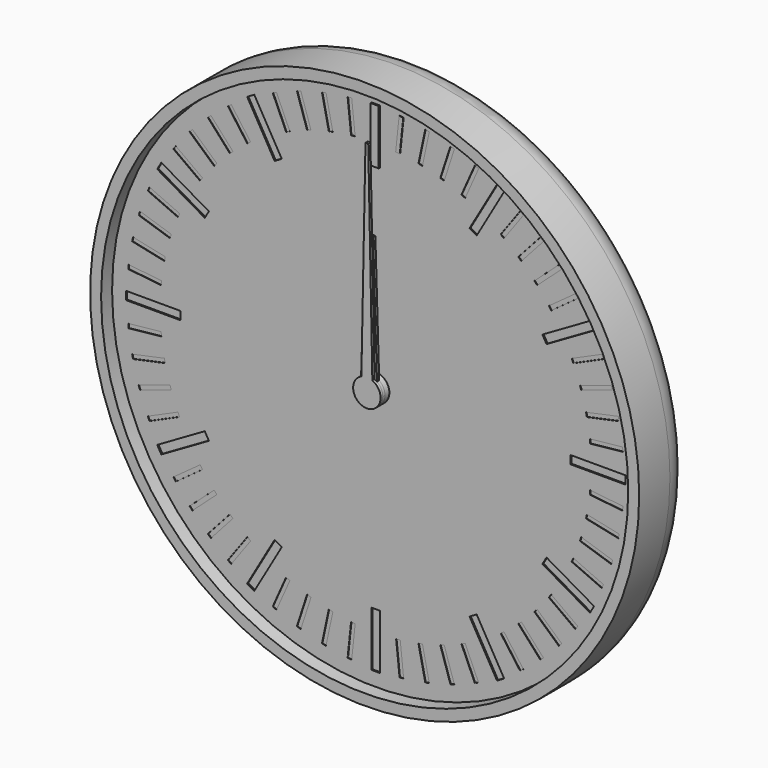
from build123d import *

# Parameters (mm, degrees)
F0_R      = 100
F1_DEPTH  = 24
F2_R      = 10
F3_T      = -4
F4_R      = 5
F4_R_2    = 3
F5_DEPTH  = 2
F6_DEPTH  = 19
F7_DEPTH  = 8
F9_DEPTH  = 4
F11_DEPTH = 4
F12_R     = 5
F12_R_2   = 3
F13_DEPTH = 2
F14_R     = 3
F15_DEPTH = 4
F17_DEPTH = 4
F18_R     = 3
F19_DEPTH = 2
F20_R     = 98
F20_R_2   = 5
F21_DEPTH = 1
F23_R     = 5
F23_R_2   = 3
F24_DEPTH = 2
F25_W     = 3
F25_H     = 20
F25_W_2   = 20
F25_H_2   = 3
F26_DEPTH = 0.5
F27_W     = 1.5
F27_H     = 12
F27_W_2   = 12
F27_H_2   = 1.5
F28_DEPTH = 0.2
F29_DEPTH = 1
F30_DEPTH = 0.4
F31_R     = 5
F31_R_2   = 3
F32_DEPTH = 5
F33_R     = 3
F34_DEPTH = 1
F36_DEPTH = 1


with BuildPart() as f1:
    # F0 (on Front) → F1 (new body)
    with BuildSketch(Plane.XZ):
        Circle(F0_R)
    extrude(amount=F1_DEPTH)

    # F2
    f2_edges = [f1.edges().sort_by_distance(p)[0] for p in [
        (-100, 0, 0),
    ]]
    fillet(f2_edges, radius=F2_R)

    # F3
    f3_openings = [f1.faces().sort_by_distance(p)[0] for p in [
        (0, -24, 0),
    ]]
    offset(amount=F3_T, openings=f3_openings)

    # F4 (on face) → F5 (join)
    with BuildSketch(Plane.XZ.offset(4)):
        Circle(F4_R)
        Circle(F4_R_2, mode=Mode.SUBTRACT)
        with Locations((40, 0)):
            Circle(F4_R)
        with Locations((40, 0)):
            Circle(F4_R_2, mode=Mode.SUBTRACT)
    extrude(amount=F5_DEPTH)


with BuildPart() as f6:
    # F6 (new): a face of the model
    f6_faces = [f1.part.faces().sort_by_distance(p)[0] for p in [
        (0, -4, 0),
    ]]
    extrude(f6_faces, amount=F6_DEPTH)

    # F8 (on face) → F9 (join)
    with BuildSketch(Plane.XZ.offset(6)):
        with BuildLine():
            ThreePointArc((9.2729637667, -1.3794085621), (9.3494561423, -0.6915886375), (9.375, 0))
            ThreePointArc((9.375, 0), (9.3494561423, 0.6915886375), (9.2729637667, 1.3794085621))
            ThreePointArc((9.2729637667, 1.3794085621), (8.9161548403, 2.8970343223), (8.3127812852, 4.3345463782))
            ThreePointArc((8.3127812852, 4.3345463782), (7.5845343223, 5.5104867402), (6.6911892658, 6.566476316))
            ThreePointArc((6.6911892658, 6.566476316), (5.5104867402, 7.5845343223), (4.1773988938, 8.3928519278))
            ThreePointArc((4.1773988938, 8.3928519278), (2.8970343223, 8.9161548403), (1.5536078905, 9.2453733036))
            ThreePointArc((1.5536078905, 9.2453733036), (0, 9.375), (-1.5536078905, 9.2453733036))
            ThreePointArc((-1.5536078905, 9.2453733036), (-2.8970343223, 8.9161548403), (-4.1773988938, 8.3928519278))
            ThreePointArc((-4.1773988938, 8.3928519278), (-5.5104867402, 7.5845343223), (-6.6911892658, 6.566476316))
            ThreePointArc((-6.6911892658, 6.566476316), (-7.5845343223, 5.5104867402), (-8.3127812852, 4.3345463782))
            ThreePointArc((-8.3127812852, 4.3345463782), (-8.9161548403, 2.8970343223), (-9.2729637667, 1.3794085621))
            ThreePointArc((-9.2729637667, 1.3794085621), (-9.375, 0), (-9.2729637667, -1.3794085621))
            ThreePointArc((-9.2729637667, -1.3794085621), (-8.9161548403, -2.8970343223), (-8.3127812852, -4.3345463782))
            ThreePointArc((-8.3127812852, -4.3345463782), (-7.5845343223, -5.5104867402), (-6.6911892658, -6.566476316))
            ThreePointArc((-6.6911892658, -6.566476316), (-5.5104867402, -7.5845343223), (-4.1773988938, -8.3928519278))
            ThreePointArc((-4.1773988938, -8.3928519278), (-2.8970343223, -8.9161548403), (-1.5536078905, -9.2453733036))
            ThreePointArc((-1.5536078905, -9.2453733036), (0, -9.375), (1.5536078905, -9.2453733036))
            ThreePointArc((1.5536078905, -9.2453733036), (2.8970343223, -8.9161548403), (4.1773988938, -8.3928519278))
            ThreePointArc((4.1773988938, -8.3928519278), (5.5104867402, -7.5845343223), (6.6911892658, -6.566476316))
            ThreePointArc((6.6911892658, -6.566476316), (7.5845343223, -5.5104867402), (8.3127812852, -4.3345463782))
            ThreePointArc((8.3127812852, -4.3345463782), (8.9161548403, -2.8970343223), (9.2729637667, -1.3794085621))
        make_face()
        with BuildLine():
            ThreePointArc((8.3127812852, 4.3345463782), (8.9161548403, 2.8970343223), (9.2729637667, 1.3794085621))
            Line((9.2729637667, 1.3794085621), (11.1823199426, 2.3946312492))
            Line((11.1823199426, 2.3946312492), (10.8182678729, 3.515068311))
            Line((10.8182678729, 3.515068311), (10.4542158031, 4.6355053728))
            Line((10.4542158031, 4.6355053728), (8.3127812852, 4.3345463782))
        make_face()
        with BuildLine():
            Line((11.1823199426, -2.3946312492), (9.2729637667, -1.3794085621))
            ThreePointArc((9.2729637667, -1.3794085621), (8.9161548403, -2.8970343223), (8.3127812852, -4.3345463782))
            Line((8.3127812852, -4.3345463782), (10.4542158031, -4.6355053728))
            Line((10.4542158031, -4.6355053728), (10.8182678729, -3.515068311))
            Line((10.8182678729, -3.515068311), (11.1823199426, -2.3946312492))
        make_face()
        with BuildLine():
            ThreePointArc((4.1773988938, 8.3928519278), (5.5104867402, 7.5845343223), (6.6911892658, 6.566476316))
            Line((6.6911892658, 6.566476316), (7.6391579371, 8.5101001246))
            Line((7.6391579371, 8.5101001246), (6.6860572448, 9.202568311))
            Line((6.6860572448, 9.202568311), (5.7329565525, 9.8950364974))
            Line((5.7329565525, 9.8950364974), (4.1773988938, 8.3928519278))
        make_face()
        with BuildLine():
            Line((7.6391579371, -8.5101001246), (6.6911892658, -6.566476316))
            ThreePointArc((6.6911892658, -6.566476316), (5.5104867402, -7.5845343223), (4.1773988938, -8.3928519278))
            Line((4.1773988938, -8.3928519278), (5.7329565525, -9.8950364974))
            Line((5.7329565525, -9.8950364974), (6.6860572448, -9.202568311))
            Line((6.6860572448, -9.202568311), (7.6391579371, -8.5101001246))
        make_face()
        with BuildLine():
            ThreePointArc((-1.5536078905, 9.2453733036), (0, 9.375), (1.5536078905, 9.2453733036))
            Line((1.5536078905, 9.2453733036), (1.1780972451, 11.375))
            Line((1.1780972451, 11.375), (0, 11.375))
            Line((0, 11.375), (-1.1780972451, 11.375))
            Line((-1.1780972451, 11.375), (-1.5536078905, 9.2453733036))
        make_face()
        with BuildLine():
            Line((1.1780972451, -11.375), (1.5536078905, -9.2453733036))
            ThreePointArc((1.5536078905, -9.2453733036), (0, -9.375), (-1.5536078905, -9.2453733036))
            Line((-1.5536078905, -9.2453733036), (-1.1780972451, -11.375))
            Line((-1.1780972451, -11.375), (0, -11.375))
            Line((0, -11.375), (1.1780972451, -11.375))
        make_face()
        with BuildLine():
            ThreePointArc((-6.6911892658, 6.566476316), (-5.5104867402, 7.5845343223), (-4.1773988938, 8.3928519278))
            Line((-4.1773988938, 8.3928519278), (-5.7329565525, 9.8950364974))
            Line((-5.7329565525, 9.8950364974), (-6.6860572448, 9.202568311))
            Line((-6.6860572448, 9.202568311), (-7.6391579371, 8.5101001246))
            Line((-7.6391579371, 8.5101001246), (-6.6911892658, 6.566476316))
        make_face()
        with BuildLine():
            Line((-5.7329565525, -9.8950364974), (-4.1773988938, -8.3928519278))
            ThreePointArc((-4.1773988938, -8.3928519278), (-5.5104867402, -7.5845343223), (-6.6911892658, -6.566476316))
            Line((-6.6911892658, -6.566476316), (-7.6391579371, -8.5101001246))
            Line((-7.6391579371, -8.5101001246), (-6.6860572448, -9.202568311))
            Line((-6.6860572448, -9.202568311), (-5.7329565525, -9.8950364974))
        make_face()
        with BuildLine():
            ThreePointArc((-9.2729637667, 1.3794085621), (-8.9161548403, 2.8970343223), (-8.3127812852, 4.3345463782))
            Line((-8.3127812852, 4.3345463782), (-10.4542158031, 4.6355053728))
            Line((-10.4542158031, 4.6355053728), (-10.8182678729, 3.515068311))
            Line((-10.8182678729, 3.515068311), (-11.1823199426, 2.3946312492))
            Line((-11.1823199426, 2.3946312492), (-9.2729637667, 1.3794085621))
        make_face()
        with BuildLine():
            Line((-10.4542158031, -4.6355053728), (-8.3127812852, -4.3345463782))
            ThreePointArc((-8.3127812852, -4.3345463782), (-8.9161548403, -2.8970343223), (-9.2729637667, -1.3794085621))
            Line((-9.2729637667, -1.3794085621), (-11.1823199426, -2.3946312492))
            Line((-11.1823199426, -2.3946312492), (-10.8182678729, -3.515068311))
            Line((-10.8182678729, -3.515068311), (-10.4542158031, -4.6355053728))
        make_face()
    extrude(amount=F9_DEPTH)

    # F35 (on face) → F36 (join)
    with BuildSketch(Plane.XZ.offset(23)):
        with BuildLine():
            ThreePointArc((-2, 4.582575695), (-2.7386127875, -4.1833001327), (5, 0))
            ThreePointArc((5, 0), (4.1833001327, 2.7386127875), (2, 4.582575695))
            ThreePointArc((2, 4.582575695), (0, 5), (-2, 4.582575695))
        make_face()
        with BuildLine():
            ThreePointArc((-2, 4.582575695), (0, 5), (2, 4.582575695))
            Line((2, 4.582575695), (0.5, 80))
            Line((0.5, 80), (0, 80))
            Line((0, 80), (-0.5, 80))
            Line((-0.5, 80), (-2, 4.582575695))
        make_face()
    extrude(amount=-F36_DEPTH)


with BuildPart() as f7:
    # F7 (new): a face of the model
    f7_faces = [f1.part.faces().sort_by_distance(p)[0] for p in [
        (40, -4, 0),
    ]]
    extrude(f7_faces, amount=F7_DEPTH)

    # F10 (on face) → F11 (join)
    with BuildSketch(Plane.XZ.offset(6)):
        with BuildLine():
            ThreePointArc((68.0829066802, -1.5381733945), (68.1144747006, -0.7693746225), (68.125, 0))
            ThreePointArc((68.125, 0), (68.1144747006, 0.7693746225), (68.0829066802, 1.5381733945))
            ThreePointArc((68.0829066802, 1.5381733945), (67.9709283072, 2.9398630294), (67.7890320221, 4.3342039956))
            ThreePointArc((67.7890320221, 4.3342039956), (67.5104012706, 5.8475163042), (67.1494235596, 7.3433252263))
            ThreePointArc((67.1494235596, 7.3433252263), (66.7484645208, 8.6911029668), (66.280643318, 10.0171558733))
            ThreePointArc((66.280643318, 10.0171558733), (65.6934659962, 11.4394680865), (65.0293803521, 12.8275385085))
            ThreePointArc((65.0293803521, 12.8275385085), (64.3569644814, 14.0625), (63.6236643925, 15.2623099717))
            ThreePointArc((63.6236643925, 15.2623099717), (62.7536029668, 16.5314602207), (61.815433119, 17.7511268046))
            ThreePointArc((61.815433119, 17.7511268046), (60.9009482166, 18.8192983038), (59.934217974, 19.8404278876))
            ThreePointArc((59.934217974, 19.8404278876), (58.8192983038, 20.9009482166), (57.6480467764, 21.8989056799))
            ThreePointArc((57.6480467764, 21.8989056799), (56.5314602207, 22.7536029668), (55.3735505752, 23.5514238999))
            ThreePointArc((55.3735505752, 23.5514238999), (54.0625, 24.3569644814), (52.709356105, 25.0895972944))
            ThreePointArc((52.709356105, 25.0895972944), (51.4394680865, 25.6934659962), (50.1409852457, 26.2331096755))
            ThreePointArc((50.1409852457, 26.2331096755), (48.6911029668, 26.7484645208), (47.2152055856, 27.1837531139))
            ThreePointArc((47.2152055856, 27.1837531139), (45.8475163042, 27.5104012706), (44.4652101991, 27.7682826779))
            ThreePointArc((44.4652101991, 27.7682826779), (42.9398630294, 27.9709283072), (41.4057159597, 28.0898484802))
            ThreePointArc((41.4057159597, 28.0898484802), (40, 28.125), (38.5942840403, 28.0898484802))
            ThreePointArc((38.5942840403, 28.0898484802), (37.0601369706, 27.9709283072), (35.5347898009, 27.7682826779))
            ThreePointArc((35.5347898009, 27.7682826779), (34.1524836958, 27.5104012706), (32.7847944144, 27.1837531139))
            ThreePointArc((32.7847944144, 27.1837531139), (31.3088970332, 26.7484645208), (29.8590147543, 26.2331096755))
            ThreePointArc((29.8590147543, 26.2331096755), (28.5605319135, 25.6934659962), (27.290643895, 25.0895972944))
            ThreePointArc((27.290643895, 25.0895972944), (25.9375, 24.3569644814), (24.6264494248, 23.5514238999))
            ThreePointArc((24.6264494248, 23.5514238999), (23.4685397793, 22.7536029668), (22.3519532236, 21.8989056799))
            ThreePointArc((22.3519532236, 21.8989056799), (21.1807016962, 20.9009482166), (20.065782026, 19.8404278876))
            ThreePointArc((20.065782026, 19.8404278876), (19.0990517834, 18.8192983038), (18.184566881, 17.7511268046))
            ThreePointArc((18.184566881, 17.7511268046), (17.2463970332, 16.5314602207), (16.3763356075, 15.2623099717))
            ThreePointArc((16.3763356075, 15.2623099717), (15.6430355186, 14.0625), (14.9706196479, 12.8275385085))
            ThreePointArc((14.9706196479, 12.8275385085), (14.3065340038, 11.4394680865), (13.719356682, 10.0171558733))
            ThreePointArc((13.719356682, 10.0171558733), (13.2515354792, 8.6911029668), (12.8505764404, 7.3433252263))
            ThreePointArc((12.8505764404, 7.3433252263), (12.4895987294, 5.8475163042), (12.2109679779, 4.3342039956))
            ThreePointArc((12.2109679779, 4.3342039956), (12.0290716928, 2.9398630294), (11.9170933198, 1.5381733945))
            ThreePointArc((11.9170933198, 1.5381733945), (11.875, 0), (11.9170933198, -1.5381733945))
            ThreePointArc((11.9170933198, -1.5381733945), (12.0290716928, -2.9398630294), (12.2109679779, -4.3342039956))
            ThreePointArc((12.2109679779, -4.3342039956), (12.4895987294, -5.8475163042), (12.8505764404, -7.3433252263))
            ThreePointArc((12.8505764404, -7.3433252263), (13.2515354792, -8.6911029668), (13.719356682, -10.0171558733))
            ThreePointArc((13.719356682, -10.0171558733), (14.3065340038, -11.4394680865), (14.9706196479, -12.8275385085))
            ThreePointArc((14.9706196479, -12.8275385085), (15.6430355186, -14.0625), (16.3763356075, -15.2623099717))
            ThreePointArc((16.3763356075, -15.2623099717), (17.2463970332, -16.5314602207), (18.184566881, -17.7511268046))
            ThreePointArc((18.184566881, -17.7511268046), (19.0990517834, -18.8192983038), (20.065782026, -19.8404278876))
            ThreePointArc((20.065782026, -19.8404278876), (21.1807016962, -20.9009482166), (22.3519532236, -21.8989056799))
            ThreePointArc((22.3519532236, -21.8989056799), (23.4685397793, -22.7536029668), (24.6264494248, -23.5514238999))
            ThreePointArc((24.6264494248, -23.5514238999), (25.9375, -24.3569644814), (27.290643895, -25.0895972944))
            ThreePointArc((27.290643895, -25.0895972944), (28.5605319135, -25.6934659962), (29.8590147543, -26.2331096755))
            ThreePointArc((29.8590147543, -26.2331096755), (31.3088970332, -26.7484645208), (32.7847944144, -27.1837531139))
            ThreePointArc((32.7847944144, -27.1837531139), (34.1524836958, -27.5104012706), (35.5347898009, -27.7682826779))
            ThreePointArc((35.5347898009, -27.7682826779), (37.0601369706, -27.9709283072), (38.5942840403, -28.0898484802))
            ThreePointArc((38.5942840403, -28.0898484802), (40, -28.125), (41.4057159597, -28.0898484802))
            ThreePointArc((41.4057159597, -28.0898484802), (42.9398630294, -27.9709283072), (44.4652101991, -27.7682826779))
            ThreePointArc((44.4652101991, -27.7682826779), (45.8475163042, -27.5104012706), (47.2152055856, -27.1837531139))
            ThreePointArc((47.2152055856, -27.1837531139), (48.6911029668, -26.7484645208), (50.1409852457, -26.2331096755))
            ThreePointArc((50.1409852457, -26.2331096755), (51.4394680865, -25.6934659962), (52.709356105, -25.0895972944))
            ThreePointArc((52.709356105, -25.0895972944), (54.0625, -24.3569644814), (55.3735505752, -23.5514238999))
            ThreePointArc((55.3735505752, -23.5514238999), (56.5314602207, -22.7536029668), (57.6480467764, -21.8989056799))
            ThreePointArc((57.6480467764, -21.8989056799), (58.8192983038, -20.9009482166), (59.934217974, -19.8404278876))
            ThreePointArc((59.934217974, -19.8404278876), (60.9009482166, -18.8192983038), (61.815433119, -17.7511268046))
            ThreePointArc((61.815433119, -17.7511268046), (62.7536029668, -16.5314602207), (63.6236643925, -15.2623099717))
            ThreePointArc((63.6236643925, -15.2623099717), (64.3569644814, -14.0625), (65.0293803521, -12.8275385085))
            ThreePointArc((65.0293803521, -12.8275385085), (65.6934659962, -11.4394680865), (66.280643318, -10.0171558733))
            ThreePointArc((66.280643318, -10.0171558733), (66.7484645208, -8.6911029668), (67.1494235596, -7.3433252263))
            ThreePointArc((67.1494235596, -7.3433252263), (67.5104012706, -5.8475163042), (67.7890320221, -4.3342039956))
            ThreePointArc((67.7890320221, -4.3342039956), (67.9709283072, -2.9398630294), (68.0829066802, -1.5381733945))
        make_face()
        with BuildLine():
            ThreePointArc((68.0829066802, 1.5381733945), (68.1144747006, 0.7693746225), (68.125, 0))
            ThreePointArc((68.125, 0), (68.1144747006, -0.7693746225), (68.0829066802, -1.5381733945))
            Line((68.0829066802, -1.5381733945), (70.125, -1.1780972451))
            Line((70.125, -1.1780972451), (70.125, 0))
            Line((70.125, 0), (70.125, 1.1780972451))
            Line((70.125, 1.1780972451), (68.0829066802, 1.5381733945))
        make_face()
        with BuildLine():
            ThreePointArc((67.1494235596, 7.3433252263), (67.5104012706, 5.8475163042), (67.7890320221, 4.3342039956))
            Line((67.7890320221, 4.3342039956), (69.7116366623, 5.1109866922))
            Line((69.7116366623, 5.1109866922), (69.4666964721, 6.2633396859))
            Line((69.4666964721, 6.2633396859), (69.2217562819, 7.4156926796))
            Line((69.2217562819, 7.4156926796), (67.1494235596, 7.3433252263))
        make_face()
        with BuildLine():
            Line((69.7116366623, -5.1109866922), (67.7890320221, -4.3342039956))
            ThreePointArc((67.7890320221, -4.3342039956), (67.5104012706, -5.8475163042), (67.1494235596, -7.3433252263))
            Line((67.1494235596, -7.3433252263), (69.2217562819, -7.4156926796))
            Line((69.2217562819, -7.4156926796), (69.4666964721, -6.2633396859))
            Line((69.4666964721, -6.2633396859), (69.7116366623, -5.1109866922))
        make_face()
        with BuildLine():
            ThreePointArc((65.0293803521, 12.8275385085), (65.6934659962, 11.4394680865), (66.280643318, 10.0171558733))
            Line((66.280643318, 10.0171558733), (67.9997322302, 11.1766959857))
            Line((67.9997322302, 11.1766959857), (67.5205569115, 12.2529413727))
            Line((67.5205569115, 12.2529413727), (67.0413815928, 13.3291867596))
            Line((67.0413815928, 13.3291867596), (65.0293803521, 12.8275385085))
        make_face()
        with BuildLine():
            Line((67.9997322302, -11.1766959857), (66.280643318, -10.0171558733))
            ThreePointArc((66.280643318, -10.0171558733), (65.6934659962, -11.4394680865), (65.0293803521, -12.8275385085))
            Line((65.0293803521, -12.8275385085), (67.0413815928, -13.3291867596))
            Line((67.0413815928, -13.3291867596), (67.5205569115, -12.2529413727))
            Line((67.5205569115, -12.2529413727), (67.9997322302, -11.1766959857))
        make_face()
        with BuildLine():
            ThreePointArc((61.815433119, 17.7511268046), (62.7536029668, 16.5314602207), (63.6236643925, 15.2623099717))
            Line((63.6236643925, 15.2623099717), (65.064105142, 16.753930033))
            Line((65.064105142, 16.753930033), (64.3716369555, 17.7070307253))
            Line((64.3716369555, 17.7070307253), (63.6791687691, 18.6601314176))
            Line((63.6791687691, 18.6601314176), (61.815433119, 17.7511268046))
        make_face()
        with BuildLine():
            Line((65.064105142, -16.753930033), (63.6236643925, -15.2623099717))
            ThreePointArc((63.6236643925, -15.2623099717), (62.7536029668, -16.5314602207), (61.815433119, -17.7511268046))
            Line((61.815433119, -17.7511268046), (63.6791687691, -18.6601314176))
            Line((63.6791687691, -18.6601314176), (64.3716369555, -17.7070307253))
            Line((64.3716369555, -17.7070307253), (65.064105142, -16.753930033))
        make_face()
        with BuildLine():
            ThreePointArc((57.6480467764, 21.8989056799), (58.8192983038, 20.9009482166), (59.934217974, 19.8404278876))
            Line((59.934217974, 19.8404278876), (61.0330563882, 21.5989369435))
            Line((61.0330563882, 21.5989369435), (60.1575595166, 22.3872378675))
            Line((60.1575595166, 22.3872378675), (59.282062645, 23.1755387915))
            Line((59.282062645, 23.1755387915), (57.6480467764, 21.8989056799))
        make_face()
        with BuildLine():
            Line((61.0330563882, -21.5989369435), (59.934217974, -19.8404278876))
            ThreePointArc((59.934217974, -19.8404278876), (58.8192983038, -20.9009482166), (57.6480467764, -21.8989056799))
            Line((57.6480467764, -21.8989056799), (59.282062645, -23.1755387915))
            Line((59.282062645, -23.1755387915), (60.1575595166, -22.3872378675))
            Line((60.1575595166, -22.3872378675), (61.0330563882, -21.5989369435))
        make_face()
        with BuildLine():
            ThreePointArc((52.709356105, 25.0895972944), (54.0625, 24.3569644814), (55.3735505752, 23.5514238999))
            Line((55.3735505752, 23.5514238999), (56.0827621424, 25.4999666665))
            Line((56.0827621424, 25.4999666665), (55.0625, 26.089015289))
            Line((55.0625, 26.089015289), (54.0422378576, 26.6780639116))
            Line((54.0422378576, 26.6780639116), (52.709356105, 25.0895972944))
        make_face()
        with BuildLine():
            Line((56.0827621424, -25.4999666665), (55.3735505752, -23.5514238999))
            ThreePointArc((55.3735505752, -23.5514238999), (54.0625, -24.3569644814), (52.709356105, -25.0895972944))
            Line((52.709356105, -25.0895972944), (54.0422378576, -26.6780639116))
            Line((54.0422378576, -26.6780639116), (55.0625, -26.089015289))
            Line((55.0625, -26.089015289), (56.0827621424, -25.4999666665))
        make_face()
        with BuildLine():
            ThreePointArc((47.2152055856, 27.1837531139), (48.6911029668, 26.7484645208), (50.1409852457, 26.2331096755))
            Line((50.1409852457, 26.2331096755), (50.4295740173, 28.2865254836))
            Line((50.4295740173, 28.2865254836), (49.3091369555, 28.6505775534))
            Line((49.3091369555, 28.6505775534), (48.1886998938, 29.0146296232))
            Line((48.1886998938, 29.0146296232), (47.2152055856, 27.1837531139))
        make_face()
        with BuildLine():
            Line((50.4295740173, -28.2865254836), (50.1409852457, -26.2331096755))
            ThreePointArc((50.1409852457, -26.2331096755), (48.6911029668, -26.7484645208), (47.2152055856, -27.1837531139))
            Line((47.2152055856, -27.1837531139), (48.1886998938, -29.0146296232))
            Line((48.1886998938, -29.0146296232), (49.3091369555, -28.6505775534))
            Line((49.3091369555, -28.6505775534), (50.4295740173, -28.2865254836))
        make_face()
        with BuildLine():
            ThreePointArc((41.4057159597, 28.0898484802), (42.9398630294, 27.9709283072), (44.4652101991, 27.7682826779))
            Line((44.4652101991, 27.7682826779), (44.3205634611, 29.8368274034))
            Line((44.3205634611, 29.8368274034), (43.1489199559, 29.959972098))
            Line((43.1489199559, 29.959972098), (41.9772764508, 30.0831167926))
            Line((41.9772764508, 30.0831167926), (41.4057159597, 28.0898484802))
        make_face()
        with BuildLine():
            Line((44.3205634611, -29.8368274034), (44.4652101991, -27.7682826779))
            ThreePointArc((44.4652101991, -27.7682826779), (42.9398630294, -27.9709283072), (41.4057159597, -28.0898484802))
            Line((41.4057159597, -28.0898484802), (41.9772764508, -30.0831167926))
            Line((41.9772764508, -30.0831167926), (43.1489199559, -29.959972098))
            Line((43.1489199559, -29.959972098), (44.3205634611, -29.8368274034))
        make_face()
        with BuildLine():
            ThreePointArc((35.5347898009, 27.7682826779), (37.0601369706, 27.9709283072), (38.5942840403, 28.0898484802))
            Line((38.5942840403, 28.0898484802), (38.0227235492, 30.0831167926))
            Line((38.0227235492, 30.0831167926), (36.8510800441, 29.959972098))
            Line((36.8510800441, 29.959972098), (35.6794365389, 29.8368274034))
            Line((35.6794365389, 29.8368274034), (35.5347898009, 27.7682826779))
        make_face()
        with BuildLine():
            Line((38.0227235492, -30.0831167926), (38.5942840403, -28.0898484802))
            ThreePointArc((38.5942840403, -28.0898484802), (37.0601369706, -27.9709283072), (35.5347898009, -27.7682826779))
            Line((35.5347898009, -27.7682826779), (35.6794365389, -29.8368274034))
            Line((35.6794365389, -29.8368274034), (36.8510800441, -29.959972098))
            Line((36.8510800441, -29.959972098), (38.0227235492, -30.0831167926))
        make_face()
        with BuildLine():
            ThreePointArc((29.8590147543, 26.2331096755), (31.3088970332, 26.7484645208), (32.7847944144, 27.1837531139))
            Line((32.7847944144, 27.1837531139), (31.8113001062, 29.0146296232))
            Line((31.8113001062, 29.0146296232), (30.6908630445, 28.6505775534))
            Line((30.6908630445, 28.6505775534), (29.5704259827, 28.2865254836))
            Line((29.5704259827, 28.2865254836), (29.8590147543, 26.2331096755))
        make_face()
        with BuildLine():
            Line((31.8113001062, -29.0146296232), (32.7847944144, -27.1837531139))
            ThreePointArc((32.7847944144, -27.1837531139), (31.3088970332, -26.7484645208), (29.8590147543, -26.2331096755))
            Line((29.8590147543, -26.2331096755), (29.5704259827, -28.2865254836))
            Line((29.5704259827, -28.2865254836), (30.6908630445, -28.6505775534))
            Line((30.6908630445, -28.6505775534), (31.8113001062, -29.0146296232))
        make_face()
        with BuildLine():
            ThreePointArc((24.6264494248, 23.5514238999), (25.9375, 24.3569644814), (27.290643895, 25.0895972944))
            Line((27.290643895, 25.0895972944), (25.9577621424, 26.6780639116))
            Line((25.9577621424, 26.6780639116), (24.9375, 26.089015289))
            Line((24.9375, 26.089015289), (23.9172378576, 25.4999666665))
            Line((23.9172378576, 25.4999666665), (24.6264494248, 23.5514238999))
        make_face()
        with BuildLine():
            Line((25.9577621424, -26.6780639116), (27.290643895, -25.0895972944))
            ThreePointArc((27.290643895, -25.0895972944), (25.9375, -24.3569644814), (24.6264494248, -23.5514238999))
            Line((24.6264494248, -23.5514238999), (23.9172378576, -25.4999666665))
            Line((23.9172378576, -25.4999666665), (24.9375, -26.089015289))
            Line((24.9375, -26.089015289), (25.9577621424, -26.6780639116))
        make_face()
        with BuildLine():
            ThreePointArc((20.065782026, 19.8404278876), (21.1807016962, 20.9009482166), (22.3519532236, 21.8989056799))
            Line((22.3519532236, 21.8989056799), (20.717937355, 23.1755387915))
            Line((20.717937355, 23.1755387915), (19.8424404834, 22.3872378675))
            Line((19.8424404834, 22.3872378675), (18.9669436118, 21.5989369435))
            Line((18.9669436118, 21.5989369435), (20.065782026, 19.8404278876))
        make_face()
        with BuildLine():
            Line((20.717937355, -23.1755387915), (22.3519532236, -21.8989056799))
            ThreePointArc((22.3519532236, -21.8989056799), (21.1807016962, -20.9009482166), (20.065782026, -19.8404278876))
            Line((20.065782026, -19.8404278876), (18.9669436118, -21.5989369435))
            Line((18.9669436118, -21.5989369435), (19.8424404834, -22.3872378675))
            Line((19.8424404834, -22.3872378675), (20.717937355, -23.1755387915))
        make_face()
        with BuildLine():
            ThreePointArc((16.3763356075, 15.2623099717), (17.2463970332, 16.5314602207), (18.184566881, 17.7511268046))
            Line((18.184566881, 17.7511268046), (16.3208312309, 18.6601314176))
            Line((16.3208312309, 18.6601314176), (15.6283630445, 17.7070307253))
            Line((15.6283630445, 17.7070307253), (14.935894858, 16.753930033))
            Line((14.935894858, 16.753930033), (16.3763356075, 15.2623099717))
        make_face()
        with BuildLine():
            Line((16.3208312309, -18.6601314176), (18.184566881, -17.7511268046))
            ThreePointArc((18.184566881, -17.7511268046), (17.2463970332, -16.5314602207), (16.3763356075, -15.2623099717))
            Line((16.3763356075, -15.2623099717), (14.935894858, -16.753930033))
            Line((14.935894858, -16.753930033), (15.6283630445, -17.7070307253))
            Line((15.6283630445, -17.7070307253), (16.3208312309, -18.6601314176))
        make_face()
        with BuildLine():
            ThreePointArc((13.719356682, 10.0171558733), (14.3065340038, 11.4394680865), (14.9706196479, 12.8275385085))
            Line((14.9706196479, 12.8275385085), (12.9586184072, 13.3291867596))
            Line((12.9586184072, 13.3291867596), (12.4794430885, 12.2529413727))
            Line((12.4794430885, 12.2529413727), (12.0002677698, 11.1766959857))
            Line((12.0002677698, 11.1766959857), (13.719356682, 10.0171558733))
        make_face()
        with BuildLine():
            Line((12.9586184072, -13.3291867596), (14.9706196479, -12.8275385085))
            ThreePointArc((14.9706196479, -12.8275385085), (14.3065340038, -11.4394680865), (13.719356682, -10.0171558733))
            Line((13.719356682, -10.0171558733), (12.0002677698, -11.1766959857))
            Line((12.0002677698, -11.1766959857), (12.4794430885, -12.2529413727))
            Line((12.4794430885, -12.2529413727), (12.9586184072, -13.3291867596))
        make_face()
        with BuildLine():
            ThreePointArc((12.2109679779, 4.3342039956), (12.4895987294, 5.8475163042), (12.8505764404, 7.3433252263))
            Line((12.8505764404, 7.3433252263), (10.7782437181, 7.4156926796))
            Line((10.7782437181, 7.4156926796), (10.5333035279, 6.2633396859))
            Line((10.5333035279, 6.2633396859), (10.2883633377, 5.1109866922))
            Line((10.2883633377, 5.1109866922), (12.2109679779, 4.3342039956))
        make_face()
        with BuildLine():
            Line((10.7782437181, -7.4156926796), (12.8505764404, -7.3433252263))
            ThreePointArc((12.8505764404, -7.3433252263), (12.4895987294, -5.8475163042), (12.2109679779, -4.3342039956))
            Line((12.2109679779, -4.3342039956), (10.2883633377, -5.1109866922))
            Line((10.2883633377, -5.1109866922), (10.5333035279, -6.2633396859))
            Line((10.5333035279, -6.2633396859), (10.7782437181, -7.4156926796))
        make_face()
        with BuildLine():
            ThreePointArc((11.9170933198, -1.5381733945), (11.875, 0), (11.9170933198, 1.5381733945))
            Line((11.9170933198, 1.5381733945), (9.875, 1.1780972451))
            Line((9.875, 1.1780972451), (9.875, 0))
            Line((9.875, 0), (9.875, -1.1780972451))
            Line((9.875, -1.1780972451), (11.9170933198, -1.5381733945))
        make_face()
    extrude(amount=F11_DEPTH)

    # F16 (on face) → F17 (join)
    with BuildSketch(Plane.XZ.offset(12)):
        with BuildLine():
            ThreePointArc((47.4288750323, -1.0304444454), (47.4821976298, -0.5164480894), (47.5, 0))
            ThreePointArc((47.5, 0), (47.4821976298, 0.5164480894), (47.4288750323, 1.0304444454))
            ThreePointArc((47.4288750323, 1.0304444454), (47.1329238722, 2.3176274578), (46.6157661985, 3.532936117))
            ThreePointArc((46.6157661985, 3.532936117), (46.0676274578, 4.4083893922), (45.4044061018, 5.2002302532))
            ThreePointArc((45.4044061018, 5.2002302532), (44.4083893922, 6.0676274578), (43.2756595386, 6.7468551628))
            ThreePointArc((43.2756595386, 6.7468551628), (42.3176274578, 7.1329238722), (41.3156377295, 7.3837048536))
            ThreePointArc((41.3156377295, 7.3837048536), (40, 7.5), (38.6843622705, 7.3837048536))
            ThreePointArc((38.6843622705, 7.3837048536), (37.6823725422, 7.1329238722), (36.7243404614, 6.7468551628))
            ThreePointArc((36.7243404614, 6.7468551628), (35.5916106078, 6.0676274578), (34.5955938982, 5.2002302532))
            ThreePointArc((34.5955938982, 5.2002302532), (33.9323725422, 4.4083893922), (33.3842338015, 3.532936117))
            ThreePointArc((33.3842338015, 3.532936117), (32.8670761278, 2.3176274578), (32.5711249677, 1.0304444454))
            ThreePointArc((32.5711249677, 1.0304444454), (32.5, 0), (32.5711249677, -1.0304444454))
            ThreePointArc((32.5711249677, -1.0304444454), (32.8670761278, -2.3176274578), (33.3842338015, -3.532936117))
            ThreePointArc((33.3842338015, -3.532936117), (33.9323725422, -4.4083893922), (34.5955938982, -5.2002302532))
            ThreePointArc((34.5955938982, -5.2002302532), (35.5916106078, -6.0676274578), (36.7243404614, -6.7468551628))
            ThreePointArc((36.7243404614, -6.7468551628), (37.6823725422, -7.1329238722), (38.6843622705, -7.3837048536))
            ThreePointArc((38.6843622705, -7.3837048536), (40, -7.5), (41.3156377295, -7.3837048536))
            ThreePointArc((41.3156377295, -7.3837048536), (42.3176274578, -7.1329238722), (43.2756595386, -6.7468551628))
            ThreePointArc((43.2756595386, -6.7468551628), (44.4083893922, -6.0676274578), (45.4044061018, -5.2002302532))
            ThreePointArc((45.4044061018, -5.2002302532), (46.0676274578, -4.4083893922), (46.6157661985, -3.532936117))
            ThreePointArc((46.6157661985, -3.532936117), (47.1329238722, -2.3176274578), (47.4288750323, -1.0304444454))
        make_face()
        with BuildLine():
            ThreePointArc((46.6157661985, 3.532936117), (47.1329238722, 2.3176274578), (47.4288750323, 1.0304444454))
            Line((47.4288750323, 1.0304444454), (49.3262785606, 2.0393117971))
            Line((49.3262785606, 2.0393117971), (48.743795249, 3.832011096))
            Line((48.743795249, 3.832011096), (46.6157661985, 3.532936117))
        make_face()
        with BuildLine():
            Line((49.3262785606, -2.0393117971), (47.4288750323, -1.0304444454))
            ThreePointArc((47.4288750323, -1.0304444454), (47.1329238722, -2.3176274578), (46.6157661985, -3.532936117))
            Line((46.6157661985, -3.532936117), (48.743795249, -3.832011096))
            Line((48.743795249, -3.832011096), (49.3262785606, -2.0393117971))
        make_face()
        with BuildLine():
            ThreePointArc((43.2756595386, 6.7468551628), (44.4083893922, 6.0676274578), (45.4044061018, 5.2002302532))
            Line((45.4044061018, 5.2002302532), (46.3464404506, 7.1316868974))
            Line((46.3464404506, 7.1316868974), (44.8214793429, 8.2396359957))
            Line((44.8214793429, 8.2396359957), (43.2756595386, 6.7468551628))
        make_face()
        with BuildLine():
            Line((46.3464404506, -7.1316868974), (45.4044061018, -5.2002302532))
            ThreePointArc((45.4044061018, -5.2002302532), (44.4083893922, -6.0676274578), (43.2756595386, -6.7468551628))
            Line((43.2756595386, -6.7468551628), (44.8214793429, -8.2396359957))
            Line((44.8214793429, -8.2396359957), (46.3464404506, -7.1316868974))
        make_face()
        with BuildLine():
            ThreePointArc((38.6843622705, 7.3837048536), (40, 7.5), (41.3156377295, 7.3837048536))
            Line((41.3156377295, 7.3837048536), (40.9424777961, 9.5))
            Line((40.9424777961, 9.5), (39.0575222039, 9.5))
            Line((39.0575222039, 9.5), (38.6843622705, 7.3837048536))
        make_face()
        with BuildLine():
            Line((40.9424777961, -9.5), (41.3156377295, -7.3837048536))
            ThreePointArc((41.3156377295, -7.3837048536), (40, -7.5), (38.6843622705, -7.3837048536))
            Line((38.6843622705, -7.3837048536), (39.0575222039, -9.5))
            Line((39.0575222039, -9.5), (40.9424777961, -9.5))
        make_face()
        with BuildLine():
            ThreePointArc((34.5955938982, 5.2002302532), (35.5916106078, 6.0676274578), (36.7243404614, 6.7468551628))
            Line((36.7243404614, 6.7468551628), (35.1785206571, 8.2396359957))
            Line((35.1785206571, 8.2396359957), (33.6535595494, 7.1316868974))
            Line((33.6535595494, 7.1316868974), (34.5955938982, 5.2002302532))
        make_face()
        with BuildLine():
            Line((35.1785206571, -8.2396359957), (36.7243404614, -6.7468551628))
            ThreePointArc((36.7243404614, -6.7468551628), (35.5916106078, -6.0676274578), (34.5955938982, -5.2002302532))
            Line((34.5955938982, -5.2002302532), (33.6535595494, -7.1316868974))
            Line((33.6535595494, -7.1316868974), (35.1785206571, -8.2396359957))
        make_face()
        with BuildLine():
            ThreePointArc((32.5711249677, 1.0304444454), (32.8670761278, 2.3176274578), (33.3842338015, 3.532936117))
            Line((33.3842338015, 3.532936117), (31.256204751, 3.832011096))
            Line((31.256204751, 3.832011096), (30.6737214394, 2.0393117971))
            Line((30.6737214394, 2.0393117971), (32.5711249677, 1.0304444454))
        make_face()
        with BuildLine():
            Line((31.256204751, -3.832011096), (33.3842338015, -3.532936117))
            ThreePointArc((33.3842338015, -3.532936117), (32.8670761278, -2.3176274578), (32.5711249677, -1.0304444454))
            Line((32.5711249677, -1.0304444454), (30.6737214394, -2.0393117971))
            Line((30.6737214394, -2.0393117971), (31.256204751, -3.832011096))
        make_face()
    extrude(amount=F17_DEPTH)

    # F18 (on face) → F19 (join)
    with BuildSketch(Plane.XZ.offset(16)):
        with Locations((40, 0)):
            Circle(F18_R)
    extrude(amount=F19_DEPTH)


with BuildPart() as f13:
    # F12 (on face) → F13 (new body)
    with BuildSketch(Plane.XZ.offset(10)):
        Circle(F12_R)
        Circle(F12_R_2, mode=Mode.SUBTRACT)
    extrude(amount=F13_DEPTH)

    # F14 (on face) → F15 (join)
    with BuildSketch(Plane.XZ.offset(12)):
        with BuildLine():
            ThreePointArc((29.9718156995, -1.3001014101), (29.9929530972, -0.6502034357), (30, 0))
            ThreePointArc((30, 0), (29.9929530972, 0.6502034357), (29.9718156995, 1.3001014101))
            ThreePointArc((29.9718156995, 1.3001014101), (29.907520012, 2.3537728718), (29.8061935814, 3.4045299509))
            ThreePointArc((29.8061935814, 3.4045299509), (29.6306502179, 4.6930339512), (29.3994322443, 5.9727199596))
            ThreePointArc((29.3994322443, 5.9727199596), (29.1710976119, 7.0033609157), (28.9066440563, 8.0253304855))
            ThreePointArc((28.9066440563, 8.0253304855), (28.5316954889, 9.2705098312), (28.1031371961, 10.4982703213))
            ThreePointArc((28.1031371961, 10.4982703213), (27.7163859753, 11.480502971), (27.2953170189, 12.448520749))
            ThreePointArc((27.2953170189, 12.448520749), (26.7301957257, 13.6197149922), (26.1148496411, 14.765318426))
            ThreePointArc((26.1148496411, 14.765318426), (25.5792049306, 15.6749569415), (25.0118886885, 16.5651871174))
            ThreePointArc((25.0118886885, 16.5651871174), (24.2705098312, 17.6335575688), (23.4835278178, 18.6687953878))
            ThreePointArc((23.4835278178, 18.6687953878), (22.812178968, 19.4834414499), (22.1125846489, 20.2739636023))
            ThreePointArc((22.1125846489, 20.2739636023), (21.2132034356, 21.2132034356), (20.2739636023, 22.1125846489))
            ThreePointArc((20.2739636023, 22.1125846489), (19.4834414499, 22.812178968), (18.6687953878, 23.4835278178))
            ThreePointArc((18.6687953878, 23.4835278178), (17.6335575688, 24.2705098312), (16.5651871174, 25.0118886885))
            ThreePointArc((16.5651871174, 25.0118886885), (15.6749569415, 25.5792049306), (14.765318426, 26.1148496411))
            ThreePointArc((14.765318426, 26.1148496411), (13.6197149922, 26.7301957257), (12.448520749, 27.2953170189))
            ThreePointArc((12.448520749, 27.2953170189), (11.480502971, 27.7163859753), (10.4982703213, 28.1031371961))
            ThreePointArc((10.4982703213, 28.1031371961), (9.2705098312, 28.5316954889), (8.0253304855, 28.9066440563))
            ThreePointArc((8.0253304855, 28.9066440563), (7.0033609157, 29.1710976119), (5.9727199596, 29.3994322443))
            ThreePointArc((5.9727199596, 29.3994322443), (4.6930339512, 29.6306502179), (3.4045299509, 29.8061935814))
            ThreePointArc((3.4045299509, 29.8061935814), (2.3537728718, 29.907520012), (1.3001014101, 29.9718156995))
            ThreePointArc((1.3001014101, 29.9718156995), (0, 30), (-1.3001014101, 29.9718156995))
            ThreePointArc((-1.3001014101, 29.9718156995), (-2.3537728718, 29.907520012), (-3.4045299509, 29.8061935814))
            ThreePointArc((-3.4045299509, 29.8061935814), (-4.6930339512, 29.6306502179), (-5.9727199596, 29.3994322443))
            ThreePointArc((-5.9727199596, 29.3994322443), (-7.0033609157, 29.1710976119), (-8.0253304855, 28.9066440563))
            ThreePointArc((-8.0253304855, 28.9066440563), (-9.2705098312, 28.5316954889), (-10.4982703213, 28.1031371961))
            ThreePointArc((-10.4982703213, 28.1031371961), (-11.480502971, 27.7163859753), (-12.448520749, 27.2953170189))
            ThreePointArc((-12.448520749, 27.2953170189), (-13.6197149922, 26.7301957257), (-14.765318426, 26.1148496411))
            ThreePointArc((-14.765318426, 26.1148496411), (-15.6749569415, 25.5792049306), (-16.5651871174, 25.0118886885))
            ThreePointArc((-16.5651871174, 25.0118886885), (-17.6335575688, 24.2705098312), (-18.6687953878, 23.4835278178))
            ThreePointArc((-18.6687953878, 23.4835278178), (-19.4834414499, 22.812178968), (-20.2739636023, 22.1125846489))
            ThreePointArc((-20.2739636023, 22.1125846489), (-21.2132034356, 21.2132034356), (-22.1125846489, 20.2739636023))
            ThreePointArc((-22.1125846489, 20.2739636023), (-22.812178968, 19.4834414499), (-23.4835278178, 18.6687953878))
            ThreePointArc((-23.4835278178, 18.6687953878), (-24.2705098312, 17.6335575688), (-25.0118886885, 16.5651871174))
            ThreePointArc((-25.0118886885, 16.5651871174), (-25.5792049306, 15.6749569415), (-26.1148496411, 14.765318426))
            ThreePointArc((-26.1148496411, 14.765318426), (-26.7301957257, 13.6197149922), (-27.2953170189, 12.448520749))
            ThreePointArc((-27.2953170189, 12.448520749), (-27.7163859753, 11.480502971), (-28.1031371961, 10.4982703213))
            ThreePointArc((-28.1031371961, 10.4982703213), (-28.5316954889, 9.2705098312), (-28.9066440563, 8.0253304855))
            ThreePointArc((-28.9066440563, 8.0253304855), (-29.1710976119, 7.0033609157), (-29.3994322443, 5.9727199596))
            ThreePointArc((-29.3994322443, 5.9727199596), (-29.6306502179, 4.6930339512), (-29.8061935814, 3.4045299509))
            ThreePointArc((-29.8061935814, 3.4045299509), (-29.907520012, 2.3537728718), (-29.9718156995, 1.3001014101))
            ThreePointArc((-29.9718156995, 1.3001014101), (-30, 0), (-29.9718156995, -1.3001014101))
            ThreePointArc((-29.9718156995, -1.3001014101), (-29.907520012, -2.3537728718), (-29.8061935814, -3.4045299509))
            ThreePointArc((-29.8061935814, -3.4045299509), (-29.6306502179, -4.6930339512), (-29.3994322443, -5.9727199596))
            ThreePointArc((-29.3994322443, -5.9727199596), (-29.1710976119, -7.0033609157), (-28.9066440563, -8.0253304855))
            ThreePointArc((-28.9066440563, -8.0253304855), (-28.5316954889, -9.2705098312), (-28.1031371961, -10.4982703213))
            ThreePointArc((-28.1031371961, -10.4982703213), (-27.7163859753, -11.480502971), (-27.2953170189, -12.448520749))
            ThreePointArc((-27.2953170189, -12.448520749), (-26.7301957257, -13.6197149922), (-26.1148496411, -14.765318426))
            ThreePointArc((-26.1148496411, -14.765318426), (-25.5792049306, -15.6749569415), (-25.0118886885, -16.5651871174))
            ThreePointArc((-25.0118886885, -16.5651871174), (-24.2705098312, -17.6335575688), (-23.4835278178, -18.6687953878))
            ThreePointArc((-23.4835278178, -18.6687953878), (-22.812178968, -19.4834414499), (-22.1125846489, -20.2739636023))
            ThreePointArc((-22.1125846489, -20.2739636023), (-21.2132034356, -21.2132034356), (-20.2739636023, -22.1125846489))
            ThreePointArc((-20.2739636023, -22.1125846489), (-19.4834414499, -22.812178968), (-18.6687953878, -23.4835278178))
            ThreePointArc((-18.6687953878, -23.4835278178), (-17.6335575688, -24.2705098312), (-16.5651871174, -25.0118886885))
            ThreePointArc((-16.5651871174, -25.0118886885), (-15.6749569415, -25.5792049306), (-14.765318426, -26.1148496411))
            ThreePointArc((-14.765318426, -26.1148496411), (-13.6197149922, -26.7301957257), (-12.448520749, -27.2953170189))
            ThreePointArc((-12.448520749, -27.2953170189), (-11.480502971, -27.7163859753), (-10.4982703213, -28.1031371961))
            ThreePointArc((-10.4982703213, -28.1031371961), (-9.2705098312, -28.5316954889), (-8.0253304855, -28.9066440563))
            ThreePointArc((-8.0253304855, -28.9066440563), (-7.0033609157, -29.1710976119), (-5.9727199596, -29.3994322443))
            ThreePointArc((-5.9727199596, -29.3994322443), (-4.6930339512, -29.6306502179), (-3.4045299509, -29.8061935814))
            ThreePointArc((-3.4045299509, -29.8061935814), (-2.3537728718, -29.907520012), (-1.3001014101, -29.9718156995))
            ThreePointArc((-1.3001014101, -29.9718156995), (0, -30), (1.3001014101, -29.9718156995))
            ThreePointArc((1.3001014101, -29.9718156995), (2.3537728718, -29.907520012), (3.4045299509, -29.8061935814))
            ThreePointArc((3.4045299509, -29.8061935814), (4.6930339512, -29.6306502179), (5.9727199596, -29.3994322443))
            ThreePointArc((5.9727199596, -29.3994322443), (7.0033609157, -29.1710976119), (8.0253304855, -28.9066440563))
            ThreePointArc((8.0253304855, -28.9066440563), (9.2705098312, -28.5316954889), (10.4982703213, -28.1031371961))
            ThreePointArc((10.4982703213, -28.1031371961), (11.480502971, -27.7163859753), (12.448520749, -27.2953170189))
            ThreePointArc((12.448520749, -27.2953170189), (13.6197149922, -26.7301957257), (14.765318426, -26.1148496411))
            ThreePointArc((14.765318426, -26.1148496411), (15.6749569415, -25.5792049306), (16.5651871174, -25.0118886885))
            ThreePointArc((16.5651871174, -25.0118886885), (17.6335575688, -24.2705098312), (18.6687953878, -23.4835278178))
            ThreePointArc((18.6687953878, -23.4835278178), (19.4834414499, -22.812178968), (20.2739636023, -22.1125846489))
            ThreePointArc((20.2739636023, -22.1125846489), (21.2132034356, -21.2132034356), (22.1125846489, -20.2739636023))
            ThreePointArc((22.1125846489, -20.2739636023), (22.812178968, -19.4834414499), (23.4835278178, -18.6687953878))
            ThreePointArc((23.4835278178, -18.6687953878), (24.2705098312, -17.6335575688), (25.0118886885, -16.5651871174))
            ThreePointArc((25.0118886885, -16.5651871174), (25.5792049306, -15.6749569415), (26.1148496411, -14.765318426))
            ThreePointArc((26.1148496411, -14.765318426), (26.7301957257, -13.6197149922), (27.2953170189, -12.448520749))
            ThreePointArc((27.2953170189, -12.448520749), (27.7163859753, -11.480502971), (28.1031371961, -10.4982703213))
            ThreePointArc((28.1031371961, -10.4982703213), (28.5316954889, -9.2705098312), (28.9066440563, -8.0253304855))
            ThreePointArc((28.9066440563, -8.0253304855), (29.1710976119, -7.0033609157), (29.3994322443, -5.9727199596))
            ThreePointArc((29.3994322443, -5.9727199596), (29.6306502179, -4.6930339512), (29.8061935814, -3.4045299509))
            ThreePointArc((29.8061935814, -3.4045299509), (29.907520012, -2.3537728718), (29.9718156995, -1.3001014101))
        make_face()
        Circle(F14_R, mode=Mode.SUBTRACT)
        with BuildLine():
            ThreePointArc((29.9718156995, 1.3001014101), (29.9929530972, 0.6502034357), (30, 0))
            ThreePointArc((30, 0), (29.9929530972, -0.6502034357), (29.9718156995, -1.3001014101))
            Line((29.9718156995, -1.3001014101), (32, -0.9424777961))
            Line((32, -0.9424777961), (32, 0))
            Line((32, 0), (32, 0.9424777961))
            Line((32, 0.9424777961), (29.9718156995, 1.3001014101))
        make_face()
        with BuildLine():
            ThreePointArc((29.3994322443, 5.9727199596), (29.6306502179, 4.6930339512), (29.8061935814, 3.4045299509))
            Line((29.8061935814, 3.4045299509), (31.7534629089, 4.0750285508))
            Line((31.7534629089, 4.0750285508), (31.606026899, 5.0059028813))
            Line((31.606026899, 5.0059028813), (31.4585908892, 5.9367772117))
            Line((31.4585908892, 5.9367772117), (29.3994322443, 5.9727199596))
        make_face()
        with BuildLine():
            Line((31.7534629089, -4.0750285508), (29.8061935814, -3.4045299509))
            ThreePointArc((29.8061935814, -3.4045299509), (29.6306502179, -4.6930339512), (29.3994322443, -5.9727199596))
            Line((29.3994322443, -5.9727199596), (31.4585908892, -5.9367772117))
            Line((31.4585908892, -5.9367772117), (31.606026899, -5.0059028813))
            Line((31.606026899, -5.0059028813), (31.7534629089, -4.0750285508))
        make_face()
        with BuildLine():
            ThreePointArc((28.1031371961, 10.4982703213), (28.5316954889, 9.2705098312), (28.9066440563, 8.0253304855))
            Line((28.9066440563, 8.0253304855), (30.7250501773, 8.9921941706))
            Line((30.7250501773, 8.9921941706), (30.4338085214, 9.88854382))
            Line((30.4338085214, 9.88854382), (30.1425668656, 10.7848934694))
            Line((30.1425668656, 10.7848934694), (28.1031371961, 10.4982703213))
        make_face()
        with BuildLine():
            Line((30.7250501773, -8.9921941706), (28.9066440563, -8.0253304855))
            ThreePointArc((28.9066440563, -8.0253304855), (28.5316954889, -9.2705098312), (28.1031371961, -10.4982703213))
            Line((28.1031371961, -10.4982703213), (30.1425668656, -10.7848934694))
            Line((30.1425668656, -10.7848934694), (30.4338085214, -9.88854382))
            Line((30.4338085214, -9.88854382), (30.7250501773, -8.9921941706))
        make_face()
        with BuildLine():
            ThreePointArc((26.1148496411, 14.765318426), (26.7301957257, 13.6197149922), (27.2953170189, 12.448520749))
            Line((27.2953170189, 12.448520749), (28.9400847397, 13.6879421265))
            Line((28.9400847397, 13.6879421265), (28.512208774, 14.5276959917))
            Line((28.512208774, 14.5276959917), (28.0843328084, 15.3674498569))
            Line((28.0843328084, 15.3674498569), (26.1148496411, 14.765318426))
        make_face()
        with BuildLine():
            Line((28.9400847397, -13.6879421265), (27.2953170189, -12.448520749))
            ThreePointArc((27.2953170189, -12.448520749), (26.7301957257, -13.6197149922), (26.1148496411, -14.765318426))
            Line((26.1148496411, -14.765318426), (28.0843328084, -15.3674498569))
            Line((28.0843328084, -15.3674498569), (28.512208774, -14.5276959917))
            Line((28.512208774, -14.5276959917), (28.9400847397, -13.6879421265))
        make_face()
        with BuildLine():
            ThreePointArc((23.4835278178, 18.6687953878), (24.2705098312, 17.6335575688), (25.0118886885, 16.5651871174))
            Line((25.0118886885, 16.5651871174), (26.4425183691, 18.0466475195))
            Line((26.4425183691, 18.0466475195), (25.88854382, 18.8091280734))
            Line((25.88854382, 18.8091280734), (25.3345692709, 19.5716086272))
            Line((25.3345692709, 19.5716086272), (23.4835278178, 18.6687953878))
        make_face()
        with BuildLine():
            Line((26.4425183691, -18.0466475195), (25.0118886885, -16.5651871174))
            ThreePointArc((25.0118886885, -16.5651871174), (24.2705098312, -17.6335575688), (23.4835278178, -18.6687953878))
            Line((23.4835278178, -18.6687953878), (25.3345692709, -19.5716086272))
            Line((25.3345692709, -19.5716086272), (25.88854382, -18.8091280734))
            Line((25.88854382, -18.8091280734), (26.4425183691, -18.0466475195))
        make_face()
        with BuildLine():
            ThreePointArc((20.2739636023, 22.1125846489), (21.2132034356, 21.2132034356), (22.1125846489, 20.2739636023))
            Line((22.1125846489, 20.2739636023), (23.2938494387, 21.9609845572))
            Line((23.2938494387, 21.9609845572), (22.627416998, 22.627416998))
            Line((22.627416998, 22.627416998), (21.9609845572, 23.2938494387))
            Line((21.9609845572, 23.2938494387), (20.2739636023, 22.1125846489))
        make_face()
        with BuildLine():
            Line((23.2938494387, -21.9609845572), (22.1125846489, -20.2739636023))
            ThreePointArc((22.1125846489, -20.2739636023), (21.2132034356, -21.2132034356), (20.2739636023, -22.1125846489))
            Line((20.2739636023, -22.1125846489), (21.9609845572, -23.2938494387))
            Line((21.9609845572, -23.2938494387), (22.627416998, -22.627416998))
            Line((22.627416998, -22.627416998), (23.2938494387, -21.9609845572))
        make_face()
        with BuildLine():
            ThreePointArc((16.5651871174, 25.0118886885), (17.6335575688, 24.2705098312), (18.6687953878, 23.4835278178))
            Line((18.6687953878, 23.4835278178), (19.5716086272, 25.3345692709))
            Line((19.5716086272, 25.3345692709), (18.8091280734, 25.88854382))
            Line((18.8091280734, 25.88854382), (18.0466475195, 26.4425183691))
            Line((18.0466475195, 26.4425183691), (16.5651871174, 25.0118886885))
        make_face()
        with BuildLine():
            Line((19.5716086272, -25.3345692709), (18.6687953878, -23.4835278178))
            ThreePointArc((18.6687953878, -23.4835278178), (17.6335575688, -24.2705098312), (16.5651871174, -25.0118886885))
            Line((16.5651871174, -25.0118886885), (18.0466475195, -26.4425183691))
            Line((18.0466475195, -26.4425183691), (18.8091280734, -25.88854382))
            Line((18.8091280734, -25.88854382), (19.5716086272, -25.3345692709))
        make_face()
        with BuildLine():
            ThreePointArc((12.448520749, 27.2953170189), (13.6197149922, 26.7301957257), (14.765318426, 26.1148496411))
            Line((14.765318426, 26.1148496411), (15.3674498569, 28.0843328084))
            Line((15.3674498569, 28.0843328084), (14.5276959917, 28.512208774))
            Line((14.5276959917, 28.512208774), (13.6879421265, 28.9400847397))
            Line((13.6879421265, 28.9400847397), (12.448520749, 27.2953170189))
        make_face()
        with BuildLine():
            Line((15.3674498569, -28.0843328084), (14.765318426, -26.1148496411))
            ThreePointArc((14.765318426, -26.1148496411), (13.6197149922, -26.7301957257), (12.448520749, -27.2953170189))
            Line((12.448520749, -27.2953170189), (13.6879421265, -28.9400847397))
            Line((13.6879421265, -28.9400847397), (14.5276959917, -28.512208774))
            Line((14.5276959917, -28.512208774), (15.3674498569, -28.0843328084))
        make_face()
        with BuildLine():
            ThreePointArc((8.0253304855, 28.9066440563), (9.2705098312, 28.5316954889), (10.4982703213, 28.1031371961))
            Line((10.4982703213, 28.1031371961), (10.7848934694, 30.1425668656))
            Line((10.7848934694, 30.1425668656), (9.88854382, 30.4338085214))
            Line((9.88854382, 30.4338085214), (8.9921941706, 30.7250501773))
            Line((8.9921941706, 30.7250501773), (8.0253304855, 28.9066440563))
        make_face()
        with BuildLine():
            Line((10.7848934694, -30.1425668656), (10.4982703213, -28.1031371961))
            ThreePointArc((10.4982703213, -28.1031371961), (9.2705098312, -28.5316954889), (8.0253304855, -28.9066440563))
            Line((8.0253304855, -28.9066440563), (8.9921941706, -30.7250501773))
            Line((8.9921941706, -30.7250501773), (9.88854382, -30.4338085214))
            Line((9.88854382, -30.4338085214), (10.7848934694, -30.1425668656))
        make_face()
        with BuildLine():
            ThreePointArc((3.4045299509, 29.8061935814), (4.6930339512, 29.6306502179), (5.9727199596, 29.3994322443))
            Line((5.9727199596, 29.3994322443), (5.9367772117, 31.4585908892))
            Line((5.9367772117, 31.4585908892), (5.0059028813, 31.606026899))
            Line((5.0059028813, 31.606026899), (4.0750285508, 31.7534629089))
            Line((4.0750285508, 31.7534629089), (3.4045299509, 29.8061935814))
        make_face()
        with BuildLine():
            Line((5.9367772117, -31.4585908892), (5.9727199596, -29.3994322443))
            ThreePointArc((5.9727199596, -29.3994322443), (4.6930339512, -29.6306502179), (3.4045299509, -29.8061935814))
            Line((3.4045299509, -29.8061935814), (4.0750285508, -31.7534629089))
            Line((4.0750285508, -31.7534629089), (5.0059028813, -31.606026899))
            Line((5.0059028813, -31.606026899), (5.9367772117, -31.4585908892))
        make_face()
        with BuildLine():
            ThreePointArc((-1.3001014101, 29.9718156995), (0, 30), (1.3001014101, 29.9718156995))
            Line((1.3001014101, 29.9718156995), (0.9424777961, 32))
            Line((0.9424777961, 32), (0, 32))
            Line((0, 32), (-0.9424777961, 32))
            Line((-0.9424777961, 32), (-1.3001014101, 29.9718156995))
        make_face()
        with BuildLine():
            Line((0.9424777961, -32), (1.3001014101, -29.9718156995))
            ThreePointArc((1.3001014101, -29.9718156995), (0, -30), (-1.3001014101, -29.9718156995))
            Line((-1.3001014101, -29.9718156995), (-0.9424777961, -32))
            Line((-0.9424777961, -32), (0, -32))
            Line((0, -32), (0.9424777961, -32))
        make_face()
        with BuildLine():
            ThreePointArc((-5.9727199596, 29.3994322443), (-4.6930339512, 29.6306502179), (-3.4045299509, 29.8061935814))
            Line((-3.4045299509, 29.8061935814), (-4.0750285508, 31.7534629089))
            Line((-4.0750285508, 31.7534629089), (-5.0059028813, 31.606026899))
            Line((-5.0059028813, 31.606026899), (-5.9367772117, 31.4585908892))
            Line((-5.9367772117, 31.4585908892), (-5.9727199596, 29.3994322443))
        make_face()
        with BuildLine():
            Line((-4.0750285508, -31.7534629089), (-3.4045299509, -29.8061935814))
            ThreePointArc((-3.4045299509, -29.8061935814), (-4.6930339512, -29.6306502179), (-5.9727199596, -29.3994322443))
            Line((-5.9727199596, -29.3994322443), (-5.9367772117, -31.4585908892))
            Line((-5.9367772117, -31.4585908892), (-5.0059028813, -31.606026899))
            Line((-5.0059028813, -31.606026899), (-4.0750285508, -31.7534629089))
        make_face()
        with BuildLine():
            ThreePointArc((-10.4982703213, 28.1031371961), (-9.2705098312, 28.5316954889), (-8.0253304855, 28.9066440563))
            Line((-8.0253304855, 28.9066440563), (-8.9921941706, 30.7250501773))
            Line((-8.9921941706, 30.7250501773), (-9.88854382, 30.4338085214))
            Line((-9.88854382, 30.4338085214), (-10.7848934694, 30.1425668656))
            Line((-10.7848934694, 30.1425668656), (-10.4982703213, 28.1031371961))
        make_face()
        with BuildLine():
            Line((-8.9921941706, -30.7250501773), (-8.0253304855, -28.9066440563))
            ThreePointArc((-8.0253304855, -28.9066440563), (-9.2705098312, -28.5316954889), (-10.4982703213, -28.1031371961))
            Line((-10.4982703213, -28.1031371961), (-10.7848934694, -30.1425668656))
            Line((-10.7848934694, -30.1425668656), (-9.88854382, -30.4338085214))
            Line((-9.88854382, -30.4338085214), (-8.9921941706, -30.7250501773))
        make_face()
        with BuildLine():
            ThreePointArc((-14.765318426, 26.1148496411), (-13.6197149922, 26.7301957257), (-12.448520749, 27.2953170189))
            Line((-12.448520749, 27.2953170189), (-13.6879421265, 28.9400847397))
            Line((-13.6879421265, 28.9400847397), (-14.5276959917, 28.512208774))
            Line((-14.5276959917, 28.512208774), (-15.3674498569, 28.0843328084))
            Line((-15.3674498569, 28.0843328084), (-14.765318426, 26.1148496411))
        make_face()
        with BuildLine():
            Line((-13.6879421265, -28.9400847397), (-12.448520749, -27.2953170189))
            ThreePointArc((-12.448520749, -27.2953170189), (-13.6197149922, -26.7301957257), (-14.765318426, -26.1148496411))
            Line((-14.765318426, -26.1148496411), (-15.3674498569, -28.0843328084))
            Line((-15.3674498569, -28.0843328084), (-14.5276959917, -28.512208774))
            Line((-14.5276959917, -28.512208774), (-13.6879421265, -28.9400847397))
        make_face()
        with BuildLine():
            ThreePointArc((-18.6687953878, 23.4835278178), (-17.6335575688, 24.2705098312), (-16.5651871174, 25.0118886885))
            Line((-16.5651871174, 25.0118886885), (-18.0466475195, 26.4425183691))
            Line((-18.0466475195, 26.4425183691), (-18.8091280734, 25.88854382))
            Line((-18.8091280734, 25.88854382), (-19.5716086272, 25.3345692709))
            Line((-19.5716086272, 25.3345692709), (-18.6687953878, 23.4835278178))
        make_face()
        with BuildLine():
            Line((-18.0466475195, -26.4425183691), (-16.5651871174, -25.0118886885))
            ThreePointArc((-16.5651871174, -25.0118886885), (-17.6335575688, -24.2705098312), (-18.6687953878, -23.4835278178))
            Line((-18.6687953878, -23.4835278178), (-19.5716086272, -25.3345692709))
            Line((-19.5716086272, -25.3345692709), (-18.8091280734, -25.88854382))
            Line((-18.8091280734, -25.88854382), (-18.0466475195, -26.4425183691))
        make_face()
        with BuildLine():
            ThreePointArc((-22.1125846489, 20.2739636023), (-21.2132034356, 21.2132034356), (-20.2739636023, 22.1125846489))
            Line((-20.2739636023, 22.1125846489), (-21.9609845572, 23.2938494387))
            Line((-21.9609845572, 23.2938494387), (-22.627416998, 22.627416998))
            Line((-22.627416998, 22.627416998), (-23.2938494387, 21.9609845572))
            Line((-23.2938494387, 21.9609845572), (-22.1125846489, 20.2739636023))
        make_face()
        with BuildLine():
            Line((-21.9609845572, -23.2938494387), (-20.2739636023, -22.1125846489))
            ThreePointArc((-20.2739636023, -22.1125846489), (-21.2132034356, -21.2132034356), (-22.1125846489, -20.2739636023))
            Line((-22.1125846489, -20.2739636023), (-23.2938494387, -21.9609845572))
            Line((-23.2938494387, -21.9609845572), (-22.627416998, -22.627416998))
            Line((-22.627416998, -22.627416998), (-21.9609845572, -23.2938494387))
        make_face()
        with BuildLine():
            ThreePointArc((-25.0118886885, 16.5651871174), (-24.2705098312, 17.6335575688), (-23.4835278178, 18.6687953878))
            Line((-23.4835278178, 18.6687953878), (-25.3345692709, 19.5716086272))
            Line((-25.3345692709, 19.5716086272), (-25.88854382, 18.8091280734))
            Line((-25.88854382, 18.8091280734), (-26.4425183691, 18.0466475195))
            Line((-26.4425183691, 18.0466475195), (-25.0118886885, 16.5651871174))
        make_face()
        with BuildLine():
            Line((-25.3345692709, -19.5716086272), (-23.4835278178, -18.6687953878))
            ThreePointArc((-23.4835278178, -18.6687953878), (-24.2705098312, -17.6335575688), (-25.0118886885, -16.5651871174))
            Line((-25.0118886885, -16.5651871174), (-26.4425183691, -18.0466475195))
            Line((-26.4425183691, -18.0466475195), (-25.88854382, -18.8091280734))
            Line((-25.88854382, -18.8091280734), (-25.3345692709, -19.5716086272))
        make_face()
        with BuildLine():
            ThreePointArc((-27.2953170189, 12.448520749), (-26.7301957257, 13.6197149922), (-26.1148496411, 14.765318426))
            Line((-26.1148496411, 14.765318426), (-28.0843328084, 15.3674498569))
            Line((-28.0843328084, 15.3674498569), (-28.512208774, 14.5276959917))
            Line((-28.512208774, 14.5276959917), (-28.9400847397, 13.6879421265))
            Line((-28.9400847397, 13.6879421265), (-27.2953170189, 12.448520749))
        make_face()
        with BuildLine():
            Line((-28.0843328084, -15.3674498569), (-26.1148496411, -14.765318426))
            ThreePointArc((-26.1148496411, -14.765318426), (-26.7301957257, -13.6197149922), (-27.2953170189, -12.448520749))
            Line((-27.2953170189, -12.448520749), (-28.9400847397, -13.6879421265))
            Line((-28.9400847397, -13.6879421265), (-28.512208774, -14.5276959917))
            Line((-28.512208774, -14.5276959917), (-28.0843328084, -15.3674498569))
        make_face()
        with BuildLine():
            ThreePointArc((-28.9066440563, 8.0253304855), (-28.5316954889, 9.2705098312), (-28.1031371961, 10.4982703213))
            Line((-28.1031371961, 10.4982703213), (-30.1425668656, 10.7848934694))
            Line((-30.1425668656, 10.7848934694), (-30.4338085214, 9.88854382))
            Line((-30.4338085214, 9.88854382), (-30.7250501773, 8.9921941706))
            Line((-30.7250501773, 8.9921941706), (-28.9066440563, 8.0253304855))
        make_face()
        with BuildLine():
            Line((-30.1425668656, -10.7848934694), (-28.1031371961, -10.4982703213))
            ThreePointArc((-28.1031371961, -10.4982703213), (-28.5316954889, -9.2705098312), (-28.9066440563, -8.0253304855))
            Line((-28.9066440563, -8.0253304855), (-30.7250501773, -8.9921941706))
            Line((-30.7250501773, -8.9921941706), (-30.4338085214, -9.88854382))
            Line((-30.4338085214, -9.88854382), (-30.1425668656, -10.7848934694))
        make_face()
        with BuildLine():
            ThreePointArc((-29.8061935814, 3.4045299509), (-29.6306502179, 4.6930339512), (-29.3994322443, 5.9727199596))
            Line((-29.3994322443, 5.9727199596), (-31.4585908892, 5.9367772117))
            Line((-31.4585908892, 5.9367772117), (-31.606026899, 5.0059028813))
            Line((-31.606026899, 5.0059028813), (-31.7534629089, 4.0750285508))
            Line((-31.7534629089, 4.0750285508), (-29.8061935814, 3.4045299509))
        make_face()
        with BuildLine():
            Line((-31.4585908892, -5.9367772117), (-29.3994322443, -5.9727199596))
            ThreePointArc((-29.3994322443, -5.9727199596), (-29.6306502179, -4.6930339512), (-29.8061935814, -3.4045299509))
            Line((-29.8061935814, -3.4045299509), (-31.7534629089, -4.0750285508))
            Line((-31.7534629089, -4.0750285508), (-31.606026899, -5.0059028813))
            Line((-31.606026899, -5.0059028813), (-31.4585908892, -5.9367772117))
        make_face()
        with BuildLine():
            ThreePointArc((-29.9718156995, -1.3001014101), (-30, 0), (-29.9718156995, 1.3001014101))
            Line((-29.9718156995, 1.3001014101), (-32, 0.9424777961))
            Line((-32, 0.9424777961), (-32, 0))
            Line((-32, 0), (-32, -0.9424777961))
            Line((-32, -0.9424777961), (-29.9718156995, -1.3001014101))
        make_face()
    extrude(amount=F15_DEPTH)

    # F31 (on face) → F32 (join)
    with BuildSketch(Plane.XZ.offset(16)):
        Circle(F31_R)
        Circle(F31_R_2, mode=Mode.SUBTRACT)
    extrude(amount=F32_DEPTH)

    # F33 (on face) → F34 (join)
    with BuildSketch(Plane.XZ.offset(21)):
        with BuildLine():
            ThreePointArc((-2.8931766575, 4.0779319303), (-2.2950072671, -4.4421775791), (5, 0))
            ThreePointArc((5, 0), (4.4421775791, 2.2950072671), (2.8931766575, 4.0779319303))
            ThreePointArc((2.8931766575, 4.0779319303), (0, 5), (-2.8931766575, 4.0779319303))
        make_face()
        Circle(F33_R, mode=Mode.SUBTRACT)
        with BuildLine():
            ThreePointArc((-2.8931766575, 4.0779319303), (0, 5), (2.8931766575, 4.0779319303))
            Line((2.8931766575, 4.0779319303), (1.5, 50))
            Line((1.5, 50), (0, 50))
            Line((0, 50), (-1.5, 50))
            Line((-1.5, 50), (-2.8931766575, 4.0779319303))
        make_face()
    extrude(amount=F34_DEPTH)


with BuildPart() as f21:
    # F20 (on face) → F21 (new body)
    with BuildSketch(Plane.XZ.offset(18)):
        Circle(F20_R)
        Circle(F20_R_2, mode=Mode.SUBTRACT)
    extrude(amount=F21_DEPTH)


with BuildPart() as f1_1:
    add(f1.part)

    # F22: cut F21
    add(f21.part, mode=Mode.SUBTRACT)


with BuildPart() as f21_1:
    add(f21.part)

    # F23 (on face) → F24 (join, through all)
    with BuildSketch(Plane(origin=(0, -18, 0), x_dir=(-1, 0, 0), z_dir=(0, 1, 0))):
        with Locations((-40, 0)):
            Circle(F23_R)
        with Locations((-40, 0)):
            Circle(F23_R_2, mode=Mode.SUBTRACT)
    extrude(amount=F24_DEPTH)

    # F25 (on face) → F26 (cut)
    with BuildSketch(Plane.XZ.offset(19)):
        with Locations((0, 81)):
            Rectangle(F25_W, F25_H)
        Polygon((-34.2009618943, 62.2378036687), (-44.2009618943, 79.5583117444), (-46.7990381057, 78.0583117444), (-36.7990381057, 60.7378036687), align=None)
        Polygon((-60.7378036687, 36.7990381057), (-78.0583117444, 46.7990381057), (-79.5583117444, 44.2009618943), (-62.2378036687, 34.2009618943), align=None)
        with Locations((-81, 0)):
            Rectangle(F25_W_2, F25_H_2)
        Polygon((-62.2378036687, -34.2009618943), (-79.5583117444, -44.2009618943), (-78.0583117444, -46.7990381057), (-60.7378036687, -36.7990381057), align=None)
        Polygon((-36.7990381057, -60.7378036687), (-46.7990381057, -78.0583117444), (-44.2009618943, -79.5583117444), (-34.2009618943, -62.2378036687), align=None)
        with Locations((0, -81)):
            Rectangle(F25_W, F25_H)
        Polygon((34.2009618943, -62.2378036687), (44.2009618943, -79.5583117444), (46.7990381057, -78.0583117444), (36.7990381057, -60.7378036687), align=None)
        Polygon((60.7378036687, -36.7990381057), (78.0583117444, -46.7990381057), (79.5583117444, -44.2009618943), (62.2378036687, -34.2009618943), align=None)
        with Locations((81, 0)):
            Rectangle(F25_W_2, F25_H_2)
        Polygon((62.2378036687, 34.2009618943), (79.5583117444, 44.2009618943), (78.0583117444, 46.7990381057), (60.7378036687, 36.7990381057), align=None)
        Polygon((36.7990381057, 60.7378036687), (46.7990381057, 78.0583117444), (44.2009618943, 79.5583117444), (34.2009618943, 62.2378036687), align=None)
    extrude(amount=-F26_DEPTH, mode=Mode.SUBTRACT)

    # F27 (on face) → F28 (cut)
    with BuildSketch(Plane.XZ.offset(19)):
        with Locations((0, 84.5)):
            Rectangle(F27_W, F27_H)
        Polygon((-8.7139345042, 90.0826278783), (-10.2057173472, 89.9258351834), (-8.951375788, 77.991572439), (-7.459592945, 78.1483651339), align=None)
        Polygon((-18.0823973185, 88.6782916345), (-19.5496187196, 88.3664240983), (-17.0546784297, 76.6286528895), (-15.5874570286, 76.9405204257), align=None)
        Polygon((-27.2527456037, 86.3023774705), (-28.6793303782, 85.8388519789), (-24.9711264457, 74.4261737834), (-23.5445416712, 74.889699275), align=None)
        Polygon((-36.1245071051, 82.980916399), (-37.4948252916, 82.3708114343), (-32.6139855747, 71.4082659426), (-31.2436673882, 72.0183709073), align=None)
        Polygon((-44.6004809472, 78.7502990425), (-45.8995190528, 78.0002990425), (-39.8995190528, 67.6079941971), (-38.6004809472, 68.3579941971), align=None)
        Polygon((-52.5878025867, 73.6568769302), (-53.8013280783, 72.7751990517), (-46.7479050507, 63.0669951192), (-45.5343795592, 63.9486729977), align=None)
        Polygon((-59.9989612564, 67.7564546605), (-61.1136784946, 66.7527587509), (-53.0841112183, 57.8350208452), (-51.9693939801, 58.8387167547), align=None)
        Polygon((-66.7527587509, 61.1136784946), (-67.7564546605, 59.9989612564), (-58.8387167547, 51.9693939801), (-57.8350208452, 53.0841112183), align=None)
        Polygon((-72.7751990517, 53.8013280783), (-73.6568769302, 52.5878025867), (-63.9486729977, 45.5343795592), (-63.0669951192, 46.7479050507), align=None)
        Polygon((-78.0002990425, 45.8995190528), (-78.7502990425, 44.6004809472), (-68.3579941971, 38.6004809472), (-67.6079941971, 39.8995190528), align=None)
        Polygon((-82.3708114343, 37.4948252916), (-82.980916399, 36.1245071051), (-72.0183709073, 31.2436673882), (-71.4082659426, 32.6139855747), align=None)
        Polygon((-85.8388519789, 28.6793303782), (-86.3023774705, 27.2527456037), (-74.889699275, 23.5445416712), (-74.4261737834, 24.9711264457), align=None)
        Polygon((-88.3664240983, 19.5496187196), (-88.6782916345, 18.0823973185), (-76.9405204257, 15.5874570286), (-76.6286528895, 17.0546784297), align=None)
        Polygon((-89.9258351834, 10.2057173472), (-90.0826278783, 8.7139345042), (-78.1483651339, 7.459592945), (-77.991572439, 8.951375788), align=None)
        with Locations((-84.5, 0)):
            Rectangle(F27_W_2, F27_H_2)
        Polygon((-90.0826278783, -8.7139345042), (-89.9258351834, -10.2057173472), (-77.991572439, -8.951375788), (-78.1483651339, -7.459592945), align=None)
        Polygon((-88.6782916345, -18.0823973185), (-88.3664240983, -19.5496187196), (-76.6286528895, -17.0546784297), (-76.9405204257, -15.5874570286), align=None)
        Polygon((-86.3023774705, -27.2527456037), (-85.8388519789, -28.6793303782), (-74.4261737834, -24.9711264457), (-74.889699275, -23.5445416712), align=None)
        Polygon((-82.980916399, -36.1245071051), (-82.3708114343, -37.4948252916), (-71.4082659426, -32.6139855747), (-72.0183709073, -31.2436673882), align=None)
        Polygon((-78.7502990425, -44.6004809472), (-78.0002990425, -45.8995190528), (-67.6079941971, -39.8995190528), (-68.3579941971, -38.6004809472), align=None)
        Polygon((-73.6568769302, -52.5878025867), (-72.7751990517, -53.8013280783), (-63.0669951192, -46.7479050507), (-63.9486729977, -45.5343795592), align=None)
        Polygon((-67.7564546605, -59.9989612564), (-66.7527587509, -61.1136784946), (-57.8350208452, -53.0841112183), (-58.8387167547, -51.9693939801), align=None)
        Polygon((-61.1136784946, -66.7527587509), (-59.9989612564, -67.7564546605), (-51.9693939801, -58.8387167547), (-53.0841112183, -57.8350208452), align=None)
        Polygon((-53.8013280783, -72.7751990517), (-52.5878025867, -73.6568769302), (-45.5343795592, -63.9486729977), (-46.7479050507, -63.0669951192), align=None)
        Polygon((-45.8995190528, -78.0002990425), (-44.6004809472, -78.7502990425), (-38.6004809472, -68.3579941971), (-39.8995190528, -67.6079941971), align=None)
        Polygon((-37.4948252916, -82.3708114343), (-36.1245071051, -82.980916399), (-31.2436673882, -72.0183709073), (-32.6139855747, -71.4082659426), align=None)
        Polygon((-28.6793303782, -85.8388519789), (-27.2527456037, -86.3023774705), (-23.5445416712, -74.889699275), (-24.9711264457, -74.4261737834), align=None)
        Polygon((-19.5496187196, -88.3664240983), (-18.0823973185, -88.6782916345), (-15.5874570286, -76.9405204257), (-17.0546784297, -76.6286528895), align=None)
        Polygon((-10.2057173472, -89.9258351834), (-8.7139345042, -90.0826278783), (-7.459592945, -78.1483651339), (-8.951375788, -77.991572439), align=None)
        with Locations((0, -84.5)):
            Rectangle(F27_W, F27_H)
        Polygon((8.7139345042, -90.0826278783), (10.2057173472, -89.9258351834), (8.951375788, -77.991572439), (7.459592945, -78.1483651339), align=None)
        Polygon((18.0823973185, -88.6782916345), (19.5496187196, -88.3664240983), (17.0546784297, -76.6286528895), (15.5874570286, -76.9405204257), align=None)
        Polygon((27.2527456037, -86.3023774705), (28.6793303782, -85.8388519789), (24.9711264457, -74.4261737834), (23.5445416712, -74.889699275), align=None)
        Polygon((36.1245071051, -82.980916399), (37.4948252916, -82.3708114343), (32.6139855747, -71.4082659426), (31.2436673882, -72.0183709073), align=None)
        Polygon((44.6004809472, -78.7502990425), (45.8995190528, -78.0002990425), (39.8995190528, -67.6079941971), (38.6004809472, -68.3579941971), align=None)
        Polygon((52.5878025867, -73.6568769302), (53.8013280783, -72.7751990517), (46.7479050507, -63.0669951192), (45.5343795592, -63.9486729977), align=None)
        Polygon((59.9989612564, -67.7564546605), (61.1136784946, -66.7527587509), (53.0841112183, -57.8350208452), (51.9693939801, -58.8387167547), align=None)
        Polygon((66.7527587509, -61.1136784946), (67.7564546605, -59.9989612564), (58.8387167547, -51.9693939801), (57.8350208452, -53.0841112183), align=None)
        Polygon((72.7751990517, -53.8013280783), (73.6568769302, -52.5878025867), (63.9486729977, -45.5343795592), (63.0669951192, -46.7479050507), align=None)
        Polygon((78.0002990425, -45.8995190528), (78.7502990425, -44.6004809472), (68.3579941971, -38.6004809472), (67.6079941971, -39.8995190528), align=None)
        Polygon((82.3708114343, -37.4948252916), (82.980916399, -36.1245071051), (72.0183709073, -31.2436673882), (71.4082659426, -32.6139855747), align=None)
        Polygon((85.8388519789, -28.6793303782), (86.3023774705, -27.2527456037), (74.889699275, -23.5445416712), (74.4261737834, -24.9711264457), align=None)
        Polygon((88.3664240983, -19.5496187196), (88.6782916345, -18.0823973185), (76.9405204257, -15.5874570286), (76.6286528895, -17.0546784297), align=None)
        Polygon((89.9258351834, -10.2057173472), (90.0826278783, -8.7139345042), (78.1483651339, -7.459592945), (77.991572439, -8.951375788), align=None)
        with Locations((84.5, 0)):
            Rectangle(F27_W_2, F27_H_2)
        Polygon((90.0826278783, 8.7139345042), (89.9258351834, 10.2057173472), (77.991572439, 8.951375788), (78.1483651339, 7.459592945), align=None)
        Polygon((88.6782916345, 18.0823973185), (88.3664240983, 19.5496187196), (76.6286528895, 17.0546784297), (76.9405204257, 15.5874570286), align=None)
        Polygon((86.3023774705, 27.2527456037), (85.8388519789, 28.6793303782), (74.4261737834, 24.9711264457), (74.889699275, 23.5445416712), align=None)
        Polygon((82.980916399, 36.1245071051), (82.3708114343, 37.4948252916), (71.4082659426, 32.6139855747), (72.0183709073, 31.2436673882), align=None)
        Polygon((78.7502990425, 44.6004809472), (78.0002990425, 45.8995190528), (67.6079941971, 39.8995190528), (68.3579941971, 38.6004809472), align=None)
        Polygon((73.6568769302, 52.5878025867), (72.7751990517, 53.8013280783), (63.0669951192, 46.7479050507), (63.9486729977, 45.5343795592), align=None)
        Polygon((67.7564546605, 59.9989612564), (66.7527587509, 61.1136784946), (57.8350208452, 53.0841112183), (58.8387167547, 51.9693939801), align=None)
        Polygon((61.1136784946, 66.7527587509), (59.9989612564, 67.7564546605), (51.9693939801, 58.8387167547), (53.0841112183, 57.8350208452), align=None)
        Polygon((53.8013280783, 72.7751990517), (52.5878025867, 73.6568769302), (45.5343795592, 63.9486729977), (46.7479050507, 63.0669951192), align=None)
        Polygon((45.8995190528, 78.0002990425), (44.6004809472, 78.7502990425), (38.6004809472, 68.3579941971), (39.8995190528, 67.6079941971), align=None)
        Polygon((37.4948252916, 82.3708114343), (36.1245071051, 82.980916399), (31.2436673882, 72.0183709073), (32.6139855747, 71.4082659426), align=None)
        Polygon((28.6793303782, 85.8388519789), (27.2527456037, 86.3023774705), (23.5445416712, 74.889699275), (24.9711264457, 74.4261737834), align=None)
        Polygon((19.5496187196, 88.3664240983), (18.0823973185, 88.6782916345), (15.5874570286, 76.9405204257), (17.0546784297, 76.6286528895), align=None)
        Polygon((10.2057173472, 89.9258351834), (8.7139345042, 90.0826278783), (7.459592945, 78.1483651339), (8.951375788, 77.991572439), align=None)
    extrude(amount=-F28_DEPTH, mode=Mode.SUBTRACT)


with BuildPart() as f29:
    # F29 (new): a face of the model
    f29_faces = [f21_1.part.faces().sort_by_distance(p)[0] for p in [
        (0, -18.5, 81),
    ]]
    extrude(f29_faces, amount=F29_DEPTH)


with BuildPart() as f30:
    # F30 (new): a face of the model
    f30_faces = [f21_1.part.faces().sort_by_distance(p)[0] for p in [
        (8.8326551461, -18.8, 84.0371001586),
    ]]
    extrude(f30_faces, amount=F30_DEPTH)


solid = Compound([f6.part, f7.part, f13.part, f1_1.part, f21_1.part, f29.part, f30.part])
